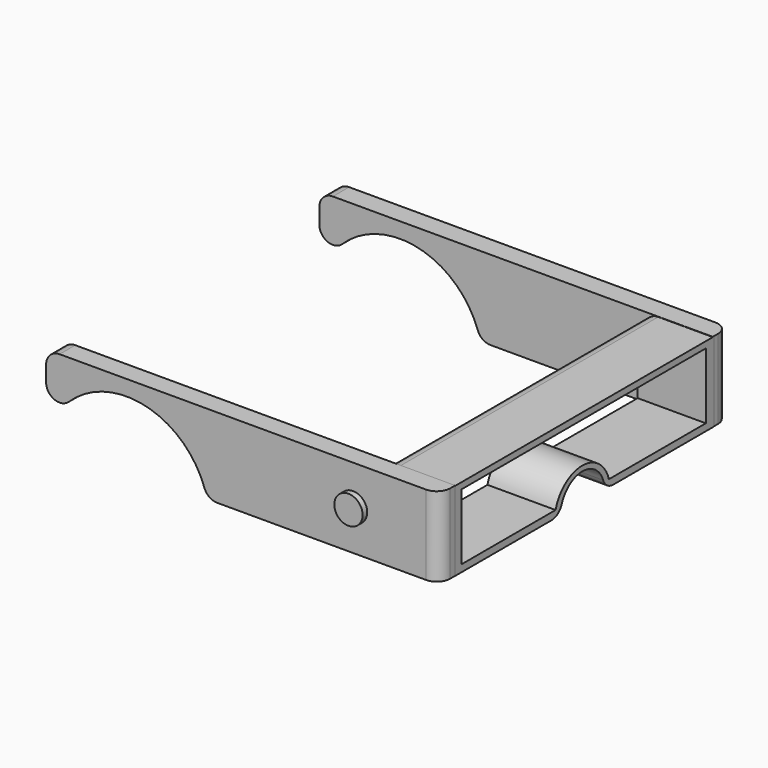
from build123d import *

# Parameters (mm, degrees)
F1_START      = 50.165
F1_DEPTH      = 7.366
F3_START      = 102.87
F3_DEPTH      = 25.654
F5_DEPTH      = 156.845
F5_DEPTH_BACK = 153.67
F7_START      = 121.285
F7_DEPTH      = 7.62
F8_R          = 5.3299304063
F9_DEPTH      = 2.159
F9_DEPTH_BACK = 3.937
F11_START     = -133.35
F10_R         = 5.3420866917
F11_DEPTH     = 7.62
F12_R         = 5.08
F13_R         = 5.08
F14_R         = 5.08
F15_T1_DEPTH  = 121.285
F16_R         = 5.08


# Not quite as in the source:
# - a fillet or chamfer that OpenCascade refuses, or shapes differently, is made with other operations: its cross-section is extruded or revolved along the edge and cut away or added


with BuildPart() as f1:
    # F0 (on Front) → F1 (new body)
    with BuildSketch(Plane.XZ.offset(F1_START)):
        with BuildLine():
            Line((128.4888833761, 0), (128.4888833761, 29.9671925604))
            Line((128.4888833761, 29.9671925604), (-19.6533282994, 29.9671925604))
            Line((-19.6533282994, 29.9671925604), (-19.6533282994, 0))
            ThreePointArc((-19.6533282994, 0), (10.6539891214, 24.1701564864), (40.9613065422, 0))
            Line((40.9613065422, 0), (128.4888833761, 0))
        make_face()
    extrude(amount=F1_DEPTH)

    # F2 (on Right) → F3 (join)
    with BuildSketch(Plane.YZ.offset(F3_START)):
        with BuildLine():
            Line((71.5717085687, 29.865141958), (-50.2199567854, 29.865141958))
            Line((-50.2199567854, 29.865141958), (-50.2199567854, 0))
            Line((-50.2199567854, 0), (-0.5977698866, 0))
            ThreePointArc((-0.5977698866, 0), (9.740347974, 10.3381178606), (20.0784658346, 0))
            Line((20.0784658346, 0), (71.5717085687, 0))
            Line((71.5717085687, 0), (71.5717085687, 29.865141958))
        make_face()
    extrude(amount=F3_DEPTH)

    # F4 (on Right) → F5 (cut, two sides)
    with BuildSketch(Plane.YZ) as f5_sk:
        with BuildLine():
            Line((67.8030401468, 27.4865683168), (-47.1380576491, 27.4865683168))
            Line((-47.1380576491, 27.4865683168), (-47.1380576491, 2.6438338682))
            Line((-47.1380576491, 2.6438338682), (-2.90596069, 2.6438338682))
            ThreePointArc((-2.90596069, 2.6438338682), (9.6324179322, 12.2636161005), (22.1707965543, 2.6438338682))
            Line((22.1707965543, 2.6438338682), (67.8030401468, 2.6438338682))
            Line((67.8030401468, 2.6438338682), (67.8030401468, 27.4865683168))
        make_face()
    extrude(amount=-F5_DEPTH, mode=Mode.SUBTRACT)
    extrude(f5_sk.sketch, amount=F5_DEPTH_BACK, mode=Mode.SUBTRACT)

    # F6 (on face) → F7 (join)
    with BuildSketch(Plane(origin=(0, -50.165, 0), x_dir=(-1, 0, 0), z_dir=(0, 1, 0)).offset(F7_START)):
        with BuildLine():
            ThreePointArc((-40.9613065422, 0), (-10.6539891214, 24.1485546437), (19.6533282994, 0))
            Line((19.6533282994, 0), (19.6533282994, 29.9671925604))
            Line((19.6533282994, 29.9671925604), (-128.4888833761, 29.9671925604))
            Line((-128.4888833761, 29.9671925604), (-128.4290701151, 0))
            Line((-128.4290701151, 0), (-40.9613065422, 0))
        make_face()
    extrude(amount=F7_DEPTH)

    # F12
    f12_edges = [f1.edges().sort_by_distance(p)[0] for p in [
        (-19.653328, -53.848, 0),
        (-19.653328, 74.93, 0),
        (-19.653328, -53.848, 29.967193),
        (-19.653328, 74.93, 29.967193),
    ]]
    fillet(f12_edges, radius=F12_R)

    # F13
    f13_edges = [f1.edges().sort_by_distance(p)[0] for p in [
        (40.961307, -53.848, 0),
        (40.961307, 74.93, 0),
    ]]
    fillet(f13_edges, radius=F13_R)

    # F14
    f14_edges = [f1.edges().sort_by_distance(p)[0] for p in [
        (115.697, -0.59777, 0),
        (115.697, 20.078466, 0),
    ]]
    fillet(f14_edges, radius=F14_R)

    # F15: fillet of radius 5.08 on 1 edges, made by hand

    # F15_s2 → F15_t1 (cut)
    with BuildSketch(Plane.XZ.offset(-71.12)):
        with BuildLine():
            ThreePointArc((102.87, 24.785141958), (104.3578975516, 28.3772444064), (107.95, 29.865141958))
            Line((107.95, 29.865141958), (102.87, 29.865141958))
            Line((102.87, 29.865141958), (102.87, 24.785141958))
        make_face()
    extrude(amount=F15_T1_DEPTH, mode=Mode.SUBTRACT)

    # F16
    f16_edges = [f1.edges().sort_by_distance(p)[0] for p in [
        (128.458977, 78.74, 14.983596),
        (128.488883, -57.531, 14.983596),
    ]]
    fillet(f16_edges, radius=F16_R)


with BuildPart() as f9:
    # F8 (on face) → F9 (new body, two sides)
    with BuildSketch(Plane.XZ.offset(57.531)) as f9_sk:
        with Locations((95.9464088082, 15.2141042054)):
            Circle(F8_R)
    extrude(amount=F9_DEPTH)
    extrude(f9_sk.sketch, amount=-F9_DEPTH_BACK)


with BuildPart() as f11:
    # F10 (on face) → F11 (new body)
    with BuildSketch(Plane.XZ.offset(59.69).offset(F11_START)):
        with Locations((95.9464088082, 15.2141042054)):
            Circle(F10_R)
    extrude(amount=-F11_DEPTH)


solid = Compound([f1.part, f9.part, f11.part])
